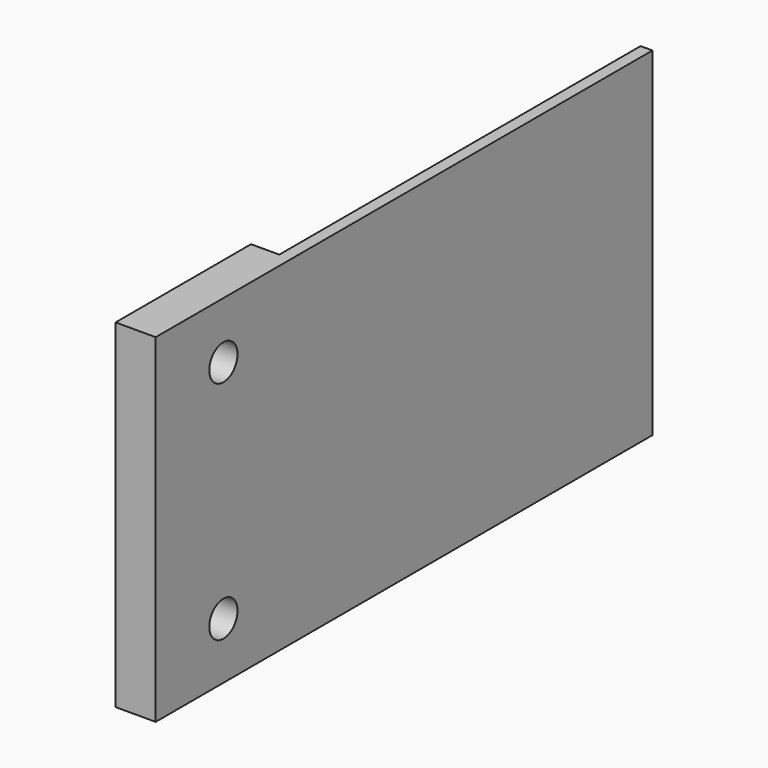
from build123d import *

# Parameters (mm, degrees)
F1_DEPTH = 38.1
F3_D     = 7.9375


# Not quite as in the source:
# - a length typed as a fraction of an inch, garbled in the dataset ("3 / 203.2 mm" for 3/8 in), is restored


with BuildPart() as f1:
    # F0 (on Top) → F1 (new body, symmetric)
    with BuildSketch(Plane.XY):
        Polygon((0, 38.1), (0, 0), (9.017, 0), (9.017, 139.7), (6.35, 139.7), (6.35, 38.1), align=None)
    extrude(amount=F1_DEPTH, both=True)

    # F3 (through all)
    with Locations(Plane.YZ.offset(9.017)):
        with Locations((19.05, 25.4), (19.05, -25.4)):
            Hole(F3_D / 2)


solid = f1.part
